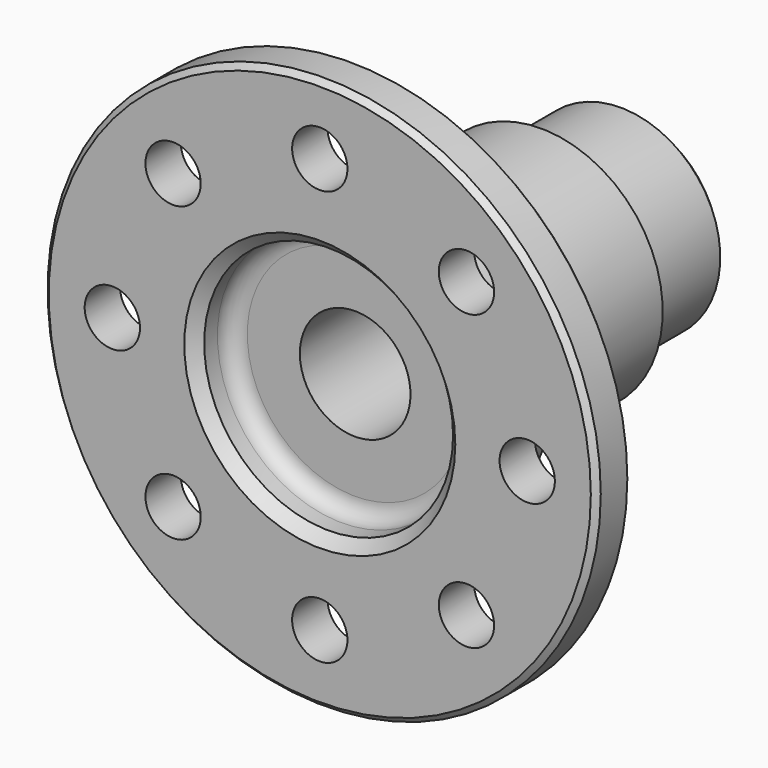
from build123d import *

# Parameters (mm, degrees)
F0_R     = 50
F0_R_2   = 5
F1_DEPTH = 8
F2_R     = 27
F3_DEPTH = 10
F4_R     = 22
F5_DEPTH = 32
F6_R     = 18
F7_DEPTH = 20
F8_R     = 22.5
F9_DEPTH = 8
F11_D    = 20
F12_SIZE = 2
F13_R    = 3
F14_SIZE = 1


with BuildPart() as f1:
    # F0 (on Front) → F1 (new body)
    with BuildSketch(Plane.XZ):
        Circle(F0_R)
        with Locations((-26.5165042945, -26.5165042945)):
            Circle(F0_R_2, mode=Mode.SUBTRACT)
        with Locations((0, -37.5)):
            Circle(F0_R_2, mode=Mode.SUBTRACT)
        with Locations((26.5165042945, -26.5165042945)):
            Circle(F0_R_2, mode=Mode.SUBTRACT)
        with Locations((-37.5, 0)):
            Circle(F0_R_2, mode=Mode.SUBTRACT)
        with Locations((-26.5165042945, 26.5165042945)):
            Circle(F0_R_2, mode=Mode.SUBTRACT)
        with Locations((37.5, 0)):
            Circle(F0_R_2, mode=Mode.SUBTRACT)
        with Locations((0, 37.5)):
            Circle(F0_R_2, mode=Mode.SUBTRACT)
        with Locations((26.5165042945, 26.5165042945)):
            Circle(F0_R_2, mode=Mode.SUBTRACT)
    extrude(amount=-F1_DEPTH)

    # F2 (on face) → F3 (join)
    with BuildSketch(Plane(origin=(0, 8, 0), x_dir=(-1, 0, 0), z_dir=(0, 1, 0))):
        Circle(F2_R)
    extrude(amount=F3_DEPTH)

    # F4 (on face) → F5 (join)
    with BuildSketch(Plane(origin=(0, 18, 0), x_dir=(-1, 0, 0), z_dir=(0, 1, 0))):
        Circle(F4_R)
    extrude(amount=F5_DEPTH)

    # F6 (on face) → F7 (join)
    with BuildSketch(Plane(origin=(0, 50, 0), x_dir=(-1, 0, 0), z_dir=(0, 1, 0))):
        Circle(F6_R)
    extrude(amount=F7_DEPTH)

    # F8 (on face) → F9 (cut)
    with BuildSketch(Plane.XZ):
        Circle(F8_R)
    extrude(amount=-F9_DEPTH, mode=Mode.SUBTRACT)

    # F11 (through all)
    with Locations(Plane.XZ.offset(-8)):
        with Locations((0, 0)):
            Hole(F11_D / 2)

    # F12
    f12_edges = [f1.edges().sort_by_distance(p)[0] for p in [
        (-22.5, 0, 0),
        (18, 70, 0),
    ]]
    chamfer(f12_edges, length=F12_SIZE)

    # F13
    f13_edges = [f1.edges().sort_by_distance(p)[0] for p in [
        (-22.5, 8, 0),
        (22, 18, 0),
        (18, 50, 0),
    ]]
    fillet(f13_edges, radius=F13_R)

    # F14
    f14_edges = [f1.edges().sort_by_distance(p)[0] for p in [
        (-50, 0, 0),
        (-50, 8, 0),
    ]]
    chamfer(f14_edges, length=F14_SIZE)


solid = f1.part
